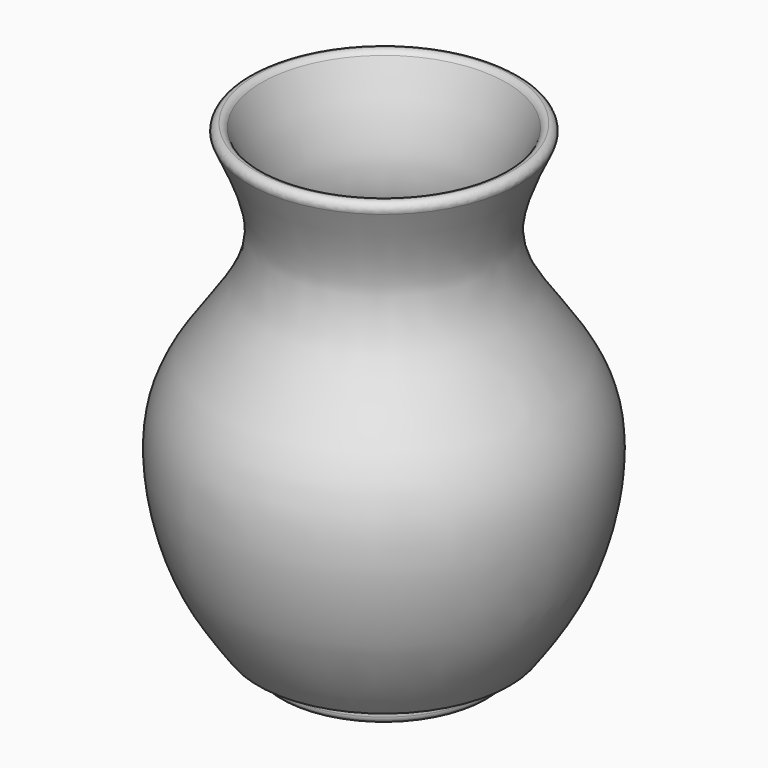
from build123d import *

# Parameters (mm, degrees)
F2_T     = -2
F3_R     = 15
F4_DEPTH = 3
F5_R     = 0.999


# Not quite as in the source:
# - a fillet or chamfer is up to 0.001 mm smaller than in the source, because OpenCascade refuses the exact size


with BuildPart() as f1:
    # F0 (on Front) → F1 (revolve)
    with BuildSketch(Plane.XZ):
        with BuildLine():
            Line((0, 65), (0, 0))
            Line((0, 0), (18, 0))
            add(Edge.make_bspline(
                [(20, 65), (17.6985697232, 60.1971369933), (13.3667166838, 51.1569775224), (19.8881851872, 40.3062857529), (28.7435315854, 29.4956838783), (25.3477464302, 10.1855330561), (20.2926354933, 3.1780784523), (18, 0)],
                knots=[0, 0, 0, 0, 0.2046672405, 0.3852336596, 0.5821458997, 0.8104913713, 1, 1, 1, 1], degree=3))
            Line((20, 65), (0, 65))
        make_face()
    revolve(axis=Axis((0, 0, 32.5), (0, 0, 1)))

    # F2
    f2_openings = [f1.faces().sort_by_distance(p)[0] for p in [
        (0, 0, 65),
    ]]
    offset(amount=F2_T, openings=f2_openings)

    # F3 (on face) → F4 (join)
    with BuildSketch(Plane(origin=(0, 0, 0), x_dir=(1, 0, 0), z_dir=(0, 0, -1))):
        Circle(F3_R)
    extrude(amount=F4_DEPTH)

    # F5 (radius 1 in the source; OpenCascade refuses exactly that, so slightly less here)
    f5_edges = [f1.edges().sort_by_distance(p)[0] for p in [
        (15, 0, -1.5),
        (-15, 0, 0),
        (-15, 0, -3),
        (-20, 0, 65),
        (-17.782713, 0, 65),
    ]]
    fillet(f5_edges, radius=F5_R)


solid = f1.part
